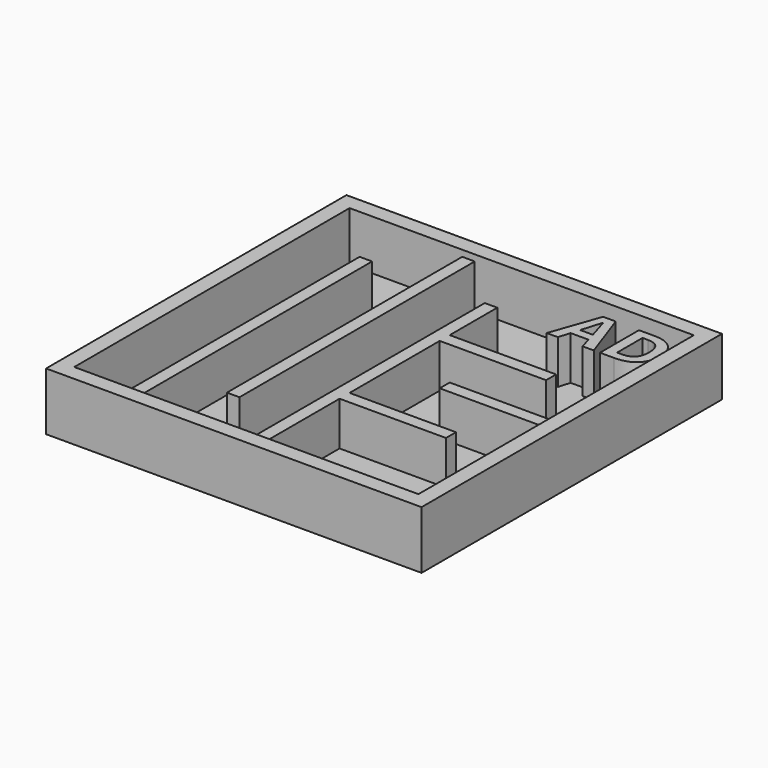
from build123d import *

# Parameters (mm, degrees)
F0_W         = 38.1
F0_H         = 38.1
F1_DEPTH     = 0.79375
F2_W         = 38.1
F2_H         = 38.1
F2_W_2       = 34.925
F2_H_2       = 34.925
F3_DEPTH     = 5.08
F4_W         = 1.27
F4_H         = 29.845
F4_W_2       = 10.795
F4_H_2       = 1.27
F5_DEPTH     = 4.445
F4_TEXT_SIZE = 6.9319154136
F6_DEPTH     = 4.445
F4_R         = 1.27
F7_DEPTH     = 0.396875


# Not quite as in the source:
# - Text() gives the source's letters only with a copy of the font that has no kerning and outlines rounded to 1/6400 em; it was checked with that copy


with BuildPart() as f1:
    # F0 (on Top) → F1 (new body)
    with BuildSketch(Plane.XY):
        with Locations((0.9983386844, -0.1242591435)):
            Rectangle(F0_W, F0_H)
    extrude(amount=F1_DEPTH)

    # F2 (on face) → F3 (join)
    with BuildSketch(Plane.XY.offset(0.79375)):
        with Locations((0.9983386844, -0.1242591435)):
            Rectangle(F2_W, F2_H)
        with Locations((0.9983386844, -0.1242591435)):
            Rectangle(F2_W_2, F2_H_2, mode=Mode.SUBTRACT)
    extrude(amount=F3_DEPTH)

    # F4 (on face) → F5 (join)
    with BuildSketch(Plane.XY.offset(0.79375)):
        with Locations((-10.7491613156, -2.6642591435)):
            Rectangle(F4_W, F4_H)
        with Locations((-4.3991613156, 2.4157408565)):
            Rectangle(F4_W, F4_H)
        Polygon((1.3158386844, 12.2582408565), (1.3158386844, -17.5867591435), (2.5858386844, -17.5867591435), (2.5858386844, -7.7442591435), (2.5858386844, -6.4742591435), (2.5858386844, 4.9557408565), (2.5858386844, 6.2257408565), (2.5858386844, 12.2582408565), align=None)
        with Locations((7.9833386844, -7.1092591435)):
            Rectangle(F4_W_2, F4_H_2)
        with Locations((7.9833386844, 5.5907408565)):
            Rectangle(F4_W_2, F4_H_2)
        with Locations((13.0633386844, -0.7592591435)):
            Rectangle(F4_W_2, F4_H_2)
    extrude(amount=F5_DEPTH)

    # F4 (on face) → F6 (join)
    with BuildSketch(Plane.XY.offset(0.79375)):
        with Locations((8.3608366549, 11.3057408565)):
            Text('AD', F4_TEXT_SIZE, font='Open Sans', font_style=FontStyle.BOLD, text_align=(TextAlign.LEFT, TextAlign.BOTTOM))
    extrude(amount=F6_DEPTH)

    # F4 (on face) → F7 (cut)
    with BuildSketch(Plane.XY.offset(0.79375)):
        with Locations((9.3247359619, -12.4041270465)):
            Circle(F4_R)
        with Locations((-13.8778015971, -14.6337337792)):
            Circle(F4_R)
    extrude(amount=-F7_DEPTH, mode=Mode.SUBTRACT)


solid = f1.part
